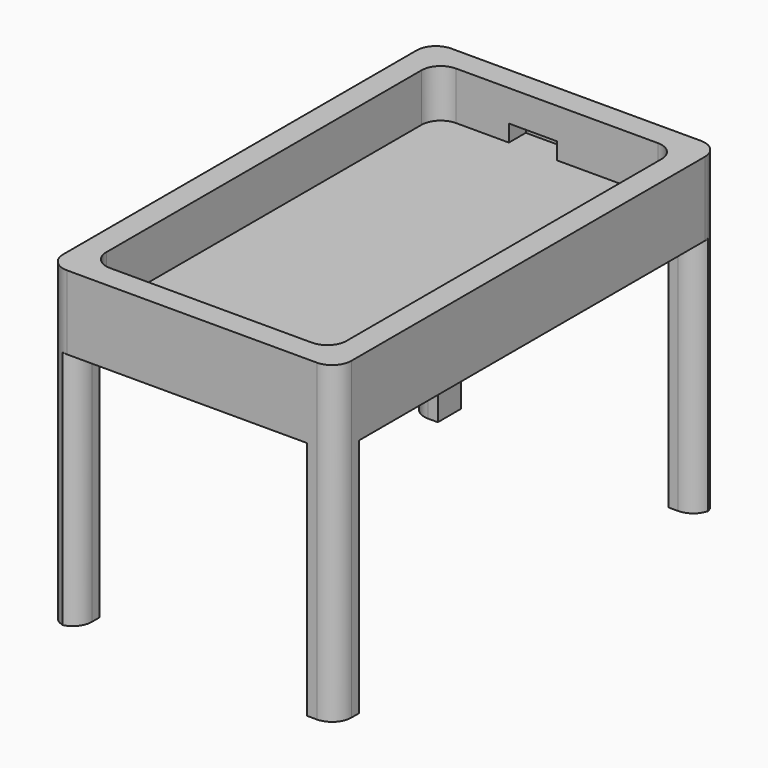
from build123d import *

# Parameters (mm, degrees)
F0_W     = 76.2
F0_H     = 127
F0_W_2   = 63.5
F0_H_2   = 114.3
F1_DEPTH = 12.7
F2_W     = 76.2
F2_H     = 127
F3_DEPTH = 6.858
F4_W     = 7.62
F4_H     = 7.62
F5_DEPTH = 63.5
F6_F1_R  = 5.08
F6_F2_R  = 5.08
F6_F3_R  = 5.08
F6_F4_R  = 5.08
F6_F5_R  = 5.08
F6_F6_R  = 5.08
F6_F7_R  = 5.08
F7_R     = 5.08
F8_W     = 12.7
F8_H     = 4.4445483945
F9_DEPTH = 5.588


with BuildPart() as f1:
    # F0 (on Top) → F1 (new body)
    with BuildSketch(Plane.XY):
        Rectangle(F0_W, F0_H)
        Rectangle(F0_W_2, F0_H_2, mode=Mode.SUBTRACT)
    extrude(amount=F1_DEPTH)

    # F2 (on Top) → F3 (join)
    with BuildSketch(Plane.XY):
        Rectangle(F2_W, F2_H)
    extrude(amount=-F3_DEPTH)

    # F4 (on face) → F5 (join)
    with BuildSketch(Plane(origin=(0, 0, -6.858), x_dir=(1, 0, 0), z_dir=(0, 0, -1))):
        with Locations((34.29, -59.69)):
            Rectangle(F4_W, F4_H)
        with Locations((34.29, 59.69)):
            Rectangle(F4_W, F4_H)
        with Locations((-34.29, 59.69)):
            Rectangle(F4_W, F4_H)
        with Locations((-34.29, -59.69)):
            Rectangle(F4_W, F4_H)
    extrude(amount=F5_DEPTH)

    # F6: fillet of radius 5.08 on 7 edges, made by hand

    # F6_f1
    f6_f1_edges = [f1.edges().sort_by_distance(p)[0] for p in [
        (38.1, 55.88, -38.608),
    ]]
    fillet(f6_f1_edges, radius=F6_F1_R)

    # F6_f2
    f6_f2_edges = [f1.edges().sort_by_distance(p)[0] for p in [
        (-38.1, 55.88, -38.608),
    ]]
    fillet(f6_f2_edges, radius=F6_F2_R)

    # F6_f3
    f6_f3_edges = [f1.edges().sort_by_distance(p)[0] for p in [
        (-30.48, -63.5, -38.608),
    ]]
    fillet(f6_f3_edges, radius=F6_F3_R)

    # F6_f4
    f6_f4_edges = [f1.edges().sort_by_distance(p)[0] for p in [
        (38.1, -63.5, -28.829),
    ]]
    fillet(f6_f4_edges, radius=F6_F4_R)

    # F6_f5
    f6_f5_edges = [f1.edges().sort_by_distance(p)[0] for p in [
        (-38.1, -63.5, -28.829),
    ]]
    fillet(f6_f5_edges, radius=F6_F5_R)

    # F6_f6
    f6_f6_edges = [f1.edges().sort_by_distance(p)[0] for p in [
        (38.1, 63.5, -28.829),
    ]]
    fillet(f6_f6_edges, radius=F6_F6_R)

    # F6_f7
    f6_f7_edges = [f1.edges().sort_by_distance(p)[0] for p in [
        (-38.1, 63.5, -28.829),
    ]]
    fillet(f6_f7_edges, radius=F6_F7_R)

    # F7
    f7_edges = [f1.edges().sort_by_distance(p)[0] for p in [
        (-31.75, -57.15, 6.35),
        (31.75, -57.15, 6.35),
        (-31.75, 57.15, 6.35),
        (31.75, 57.15, 6.35),
    ]]
    fillet(f7_edges, radius=F7_R)

    # F8 (on face) → F9 (cut)
    with BuildSketch(Plane.XZ.offset(-57.15)):
        with Locations((-6.35, 2.2222741973)):
            Rectangle(F8_W, F8_H)
    extrude(amount=-F9_DEPTH, mode=Mode.SUBTRACT)


solid = f1.part
